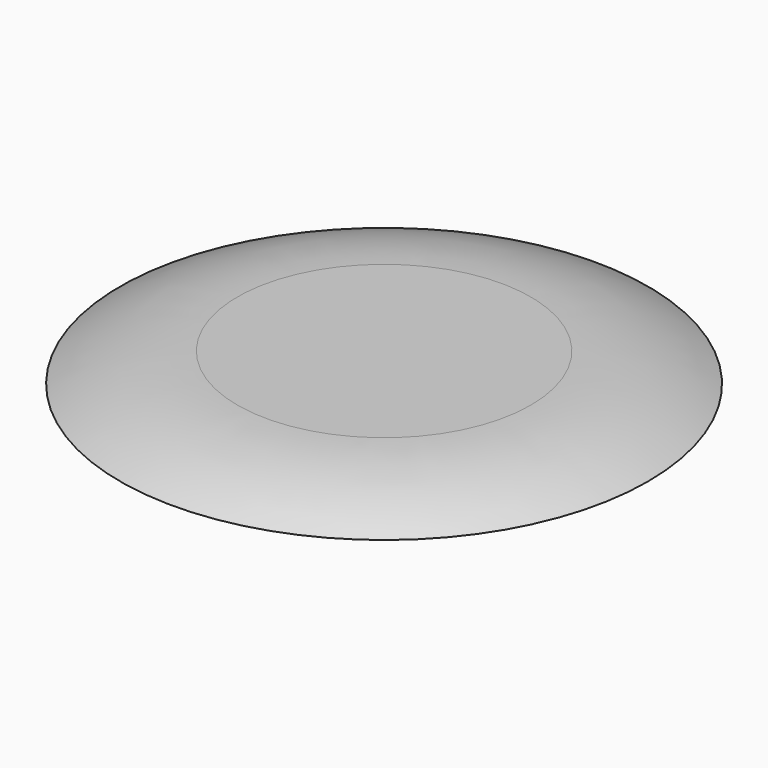
from build123d import *

# Parameters (mm, degrees)
F0_R     = 75.5041156062
F1_DEPTH = 8.2937050611
F4_T     = -2.54


# Not quite as in the source:
# - a fillet or chamfer that OpenCascade refuses, or shapes differently, is made with other operations: its cross-section is extruded or revolved along the edge and cut away or added


with BuildPart() as f1:
    # F0 (on Top) → F1 (new body)
    with BuildSketch(Plane.XY):
        Circle(F0_R)
    extrude(amount=F1_DEPTH)

    # F3: fillet of radius 72.0120994422 on 1 edges, made by hand

    # F3_s1 → F3_t2 (revolve, cut)
    with BuildSketch(Plane.XZ):
        with BuildLine():
            ThreePointArc((75.5041156062, 0), (59.2332610775, 6.189537281), (41.9525331761, 8.2937050611))
            Line((41.9525331761, 8.2937050611), (41.9525331761, 9.7339470499))
            Line((41.9525331761, 9.7339470499), (75.5041156062, 9.7339470499))
            Line((75.5041156062, 9.7339470499), (76.9443575951, 8.2937050611))
            ThreePointArc((76.9443575951, 8.2937050611), (76.9443575951, 4.1468525305), (76.1751472548, 1.2743678876))
            Line((76.1751472548, 1.2743678876), (75.5041156062, 0))
        make_face()
    revolve(axis=Axis((0, 0, 8.2937050611), (0, 0, 1)), mode=Mode.SUBTRACT)

    # F4
    f4_openings = [f1.faces().sort_by_distance(p)[0] for p in [
        (0, 0, 0),
    ]]
    offset(amount=F4_T, openings=f4_openings)


solid = f1.part
